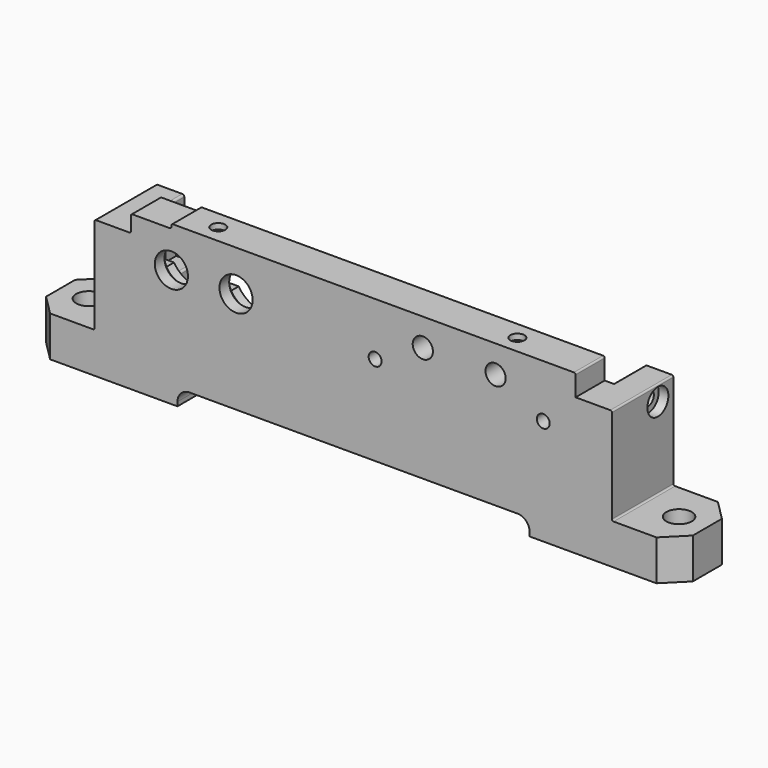
from build123d import *

# Parameters (mm, degrees)
F2_DEPTH     = 9
F3_DEPTH     = 10
F4_R         = 4.1
F4_R_2       = 2.5
F4_R_3       = 1.6
F5_DEPTH     = 24.8
F6_DEPTH     = 3
F4_R_4       = 5
F7_DEPTH     = 6
F4_R_5       = 7.75
F8_DEPTH     = 5
F9_R         = 1.75
F10_DEPTH    = 158.2
F9_R_2       = 3.25
F11_DEPTH    = 2.4
F12_R        = 3.25
F13_DEPTH    = 2.4
F14_R        = 3.4
F14_R_2      = 1.75
F15_DEPTH    = 3
F16_DEPTH    = 25
F17_W        = 100
F17_H        = 9
F18_DEPTH    = 1.1
F20_START    = -1.4
F19_R        = 1.75
F20_DEPTH    = 2.6
F21_DEPTH    = 4.2
F22_W        = 6.7549981495
F22_H        = 2.6
F23_DEPTH    = 4.5
F24_W        = 19
F24_H        = 10
F25_DEPTH    = 16
F26_SIZE     = 5
F27_W        = 19
F27_H        = 10
F28_DEPTH    = 16
F29_SIZE     = 5
F30_R        = 3.15
F31_DEPTH    = 25
F32_R        = 0.4
F33_W        = 87.1225009252
F33_H        = 9
F34_DEPTH    = 4
F35_T1_DEPTH = 9
F37_DEPTH    = 4


# Not quite as in the source:
# - a fillet or chamfer that OpenCascade refuses, or shapes differently, is made with other operations: its cross-section is extruded or revolved along the edge and cut away or added


with BuildPart() as f2:
    # F1 (on face) → F2 (new body)
    with BuildSketch(Plane.XZ):
        Polygon((-55, 28), (-64, 28), (-64, -6), (0, -6), (64, -6), (64, 28), (55, 28), (55, 32.2), (0, 32.2), (-55, 32.2), align=None)
    extrude(amount=F2_DEPTH)

    # F0 (on Front) → F3 (join)
    with BuildSketch(Plane.XZ):
        with BuildLine():
            Line((-57.5, 28), (-64, 28))
            Line((-64, 28), (-64, -6))
            Line((-64, -6), (-43.5, -6))
            Line((-43.5, -6), (-43.5, 0))
            Line((-43.5, 0), (-55, 0))
            ThreePointArc((-55, 0), (-55.3535533906, -0.1464466094), (-55.5, -0.5))
            Line((-55.5, -0.5), (-55.5, -1.5))
            Line((-55.5, -1.5), (-59, -1.5))
            Line((-59, -1.5), (-59, 6.5))
            Line((-59, 6.5), (-54.7, 6.5))
            ThreePointArc((-54.7, 6.5), (-54.3464466094, 6.6464466094), (-54.2, 7))
            Line((-54.2, 7), (-54.2, 13.5))
            ThreePointArc((-54.2, 13.5), (-54.3464466094, 13.8535533906), (-54.7, 14))
            Line((-54.7, 14), (-59, 14))
            Line((-59, 14), (-59, 20.5))
            Line((-59, 20.5), (-57.5, 20.5))
            ThreePointArc((-57.5, 20.5), (-57.1464466094, 20.6464466094), (-57, 21))
            Line((-57, 21), (-57, 27.5))
            ThreePointArc((-57, 27.5), (-57.1464466094, 27.8535533906), (-57.5, 28))
        make_face()
        with BuildLine():
            Line((43.5, -6), (64, -6))
            Line((64, -6), (64, 28))
            Line((64, 28), (57.5, 28))
            ThreePointArc((57.5, 28), (57.1464466094, 27.8535533906), (57, 27.5))
            Line((57, 27.5), (57, 21))
            ThreePointArc((57, 21), (57.1464466094, 20.6464466094), (57.5, 20.5))
            Line((57.5, 20.5), (59, 20.5))
            Line((59, 20.5), (59, 14))
            Line((59, 14), (54.7, 14))
            ThreePointArc((54.7, 14), (54.3464466094, 13.8535533906), (54.2, 13.5))
            Line((54.2, 13.5), (54.2, 7))
            ThreePointArc((54.2, 7), (54.3464466094, 6.6464466094), (54.7, 6.5))
            Line((54.7, 6.5), (59, 6.5))
            Line((59, 6.5), (59, -1.5))
            Line((59, -1.5), (55.5, -1.5))
            Line((55.5, -1.5), (55.5, -0.5))
            ThreePointArc((55.5, -0.5), (55.3535533906, -0.1464466094), (55, 0))
            Line((55, 0), (43.5, 0))
            Line((43.5, 0), (43.5, -6))
        make_face()
    extrude(amount=-F3_DEPTH)

    # F4 (on Front) → F5 (cut)
    with BuildSketch(Plane.XZ):
        with Locations((-29, 23.2)):
            Circle(F4_R)
        with Locations((-45, 23.2)):
            Circle(F4_R)
        with Locations((35.2, 26.5)):
            Circle(F4_R_2)
        with Locations((17.2, 26.5)):
            Circle(F4_R_2)
        with Locations((5.4, 20.2)):
            Circle(F4_R_3)
        with Locations((47, 20.2)):
            Circle(F4_R_3)
    extrude(amount=F5_DEPTH, mode=Mode.SUBTRACT)

    # F4 (on Front) → F6 (cut)
    with BuildSketch(Plane.XZ):
        Polygon((3.7112504626, 17.275), (7.0887495374, 17.275), (8.7774990748, 20.2), (7.0887495374, 23.125), (3.7112504626, 23.125), (2.0225009252, 20.2), align=None)
        with Locations((5.4, 20.2)):
            Circle(F4_R_3, mode=Mode.SUBTRACT)
        Polygon((45.3112504626, 17.275), (48.6887495374, 17.275), (50.3774990748, 20.2), (48.6887495374, 23.125), (45.3112504626, 23.125), (43.6225009252, 20.2), align=None)
        with Locations((47, 20.2)):
            Circle(F4_R_3, mode=Mode.SUBTRACT)
    extrude(amount=F6_DEPTH, mode=Mode.SUBTRACT)

    # F4 (on Front) → F7 (cut)
    with BuildSketch(Plane.XZ):
        with Locations((-45, 23.2)):
            Circle(F4_R_4)
        with Locations((-45, 23.2)):
            Circle(F4_R, mode=Mode.SUBTRACT)
        with Locations((-29, 23.2)):
            Circle(F4_R_4)
        with Locations((-29, 23.2)):
            Circle(F4_R, mode=Mode.SUBTRACT)
    extrude(amount=F7_DEPTH, mode=Mode.SUBTRACT)

    # F4 (on Front) → F8 (cut)
    with BuildSketch(Plane.XZ):
        with Locations((-29, 23.2)):
            Circle(F4_R_5)
        with Locations((-29, 23.2)):
            Circle(F4_R_4, mode=Mode.SUBTRACT)
        with Locations((-45, 23.2)):
            Circle(F4_R_5)
        with Locations((-45, 23.2)):
            Circle(F4_R_4, mode=Mode.SUBTRACT)
    extrude(amount=F8_DEPTH, mode=Mode.SUBTRACT)

    # F9 (on face) → F10 (cut)
    with BuildSketch(Plane(origin=(-64, 0, 0), x_dir=(0, -1, 0), z_dir=(-1, 0, 0))):
        with Locations((-5.2, 24.2)):
            Circle(F9_R)
    extrude(amount=-F10_DEPTH, mode=Mode.SUBTRACT)

    # F9 (on face) → F11 (cut)
    with BuildSketch(Plane(origin=(-64, 0, 0), x_dir=(0, -1, 0), z_dir=(-1, 0, 0))):
        with Locations((-5.2, 24.2)):
            Circle(F9_R_2)
        with Locations((-5.2, 24.2)):
            Circle(F9_R, mode=Mode.SUBTRACT)
    extrude(amount=-F11_DEPTH, mode=Mode.SUBTRACT)

    # F12 (on face) → F13 (cut)
    with BuildSketch(Plane.YZ.offset(64)):
        with Locations((5.2, 24.2)):
            Circle(F12_R)
    extrude(amount=-F13_DEPTH, mode=Mode.SUBTRACT)

    # F14 (on face) → F15 (cut)
    with BuildSketch(Plane(origin=(0, 0, -6), x_dir=(1, 0, 0), z_dir=(0, 0, -1))):
        with Locations((49.8, -5.1)):
            Circle(F14_R)
        with Locations((49.8, -5.1)):
            Circle(F14_R_2, mode=Mode.SUBTRACT)
        with Locations((-48.5, -5.1)):
            Circle(F14_R)
        with Locations((-48.5, -5.1)):
            Circle(F14_R_2, mode=Mode.SUBTRACT)
        with Locations((49.8, -5.1)):
            Circle(F14_R_2)
    extrude(amount=-F15_DEPTH, mode=Mode.SUBTRACT)

    # F14 (on face) → F16 (cut)
    with BuildSketch(Plane(origin=(0, 0, -6), x_dir=(1, 0, 0), z_dir=(0, 0, -1))):
        with Locations((49.8, -5.1)):
            Circle(F14_R_2)
        with Locations((-48.5, -5.1)):
            Circle(F14_R_2)
    extrude(amount=-F16_DEPTH, mode=Mode.SUBTRACT)

    # F17 (on face) → F18 (join)
    with BuildSketch(Plane.XY.offset(32.2)):
        with Locations((5, -4.5)):
            Rectangle(F17_W, F17_H)
    extrude(amount=F18_DEPTH)

    # F19 (on face) → F20 (cut)
    with BuildSketch(Plane.XY.offset(33.3).offset(F20_START)):
        Polygon((35.3112504626, -7.425), (38.6887495374, -7.425), (40.3774990748, -4.5), (38.6887495374, -1.575), (35.3112504626, -1.575), (33.6225009252, -4.5), align=None)
        with Locations((37, -4.5)):
            Circle(F19_R, mode=Mode.SUBTRACT)
        Polygon((-38.6887495374, -7.425), (-35.3112504626, -7.425), (-33.6225009252, -4.5), (-35.3112504626, -1.575), (-38.6887495374, -1.575), (-40.3774990748, -4.5), align=None)
        with Locations((-37, -4.5)):
            Circle(F19_R, mode=Mode.SUBTRACT)
    extrude(amount=-F20_DEPTH, mode=Mode.SUBTRACT)

    # F19 (on face) → F21 (cut)
    with BuildSketch(Plane.XY.offset(33.3)):
        with Locations((-37, -4.5)):
            Circle(F19_R)
        with Locations((37, -4.5)):
            Circle(F19_R)
    extrude(amount=-F21_DEPTH, mode=Mode.SUBTRACT)

    # F22 (on face) → F23 (cut)
    with BuildSketch(Plane(origin=(0, 0, 0), x_dir=(-1, 0, 0), z_dir=(0, 1, 0))):
        with Locations((-37, 30.6)):
            Rectangle(F22_W, F22_H)
        with Locations((37, 30.6)):
            Rectangle(F22_W, F22_H)
    extrude(amount=-F23_DEPTH, mode=Mode.SUBTRACT)

    # F24 (on face) → F25 (join)
    with BuildSketch(Plane(origin=(-64, 0, 0), x_dir=(0, -1, 0), z_dir=(-1, 0, 0))):
        with Locations((-0.5, -1)):
            Rectangle(F24_W, F24_H)
    extrude(amount=F25_DEPTH)

    # F26
    f26_edges = [f2.edges().sort_by_distance(p)[0] for p in [
        (-80, -9, -1),
        (-80, 10, -1),
    ]]
    chamfer(f26_edges, length=F26_SIZE)

    # F27 (on face) → F28 (join)
    with BuildSketch(Plane.YZ.offset(64)):
        with Locations((0.5, -1)):
            Rectangle(F27_W, F27_H)
    extrude(amount=F28_DEPTH)

    # F29
    f29_edges = [f2.edges().sort_by_distance(p)[0] for p in [
        (80, 10, -1),
        (80, -9, -1),
    ]]
    chamfer(f29_edges, length=F29_SIZE)

    # F30 (on face) → F31 (cut)
    with BuildSketch(Plane(origin=(0, 0, -6), x_dir=(1, 0, 0), z_dir=(0, 0, -1))):
        with Locations((-73, -0.5)):
            Circle(F30_R)
        with Locations((73, -0.5)):
            Circle(F30_R)
    extrude(amount=-F31_DEPTH, mode=Mode.SUBTRACT)

    # F32
    f32_edges = [f2.edges().sort_by_distance(p)[0] for p in [
        (64, 0.5, 28),
        (55, -4.5, 33.3),
        (-64, 0.5, 28),
        (-55, -4.5, 28),
        (-55, -4.5, 32.2),
        (-45, -4.5, 32.2),
        (-45, -4.5, 33.3),
        (-64, 0.5, 4),
        (64, 0.5, 4),
    ]]
    fillet(f32_edges, radius=F32_R)

    # F33 (on face) → F34 (cut)
    with BuildSketch(Plane(origin=(0, 0, -6), x_dir=(1, 0, 0), z_dir=(0, 0, -1))):
        with Locations((0.0612504626, 4.5)):
            Rectangle(F33_W, F33_H)
    extrude(amount=-F34_DEPTH, mode=Mode.SUBTRACT)

    # F35: fillet of radius 3 on 2 edges, made by hand

    # F35_s2 → F35_t1 (join)
    with BuildSketch(Plane.XZ):
        with BuildLine():
            ThreePointArc((-43.5, -5), (-42.6213203436, -2.8786796564), (-40.5, -2))
            Line((-40.5, -2), (-43.5, -2))
            Line((-43.5, -2), (-43.5, -5))
        make_face()
        with BuildLine():
            ThreePointArc((40.6225009252, -2), (42.7438212688, -2.8786796564), (43.6225009252, -5))
            Line((43.6225009252, -5), (43.6225009252, -2))
            Line((43.6225009252, -2), (40.6225009252, -2))
        make_face()
    extrude(amount=F35_T1_DEPTH)

    # F36 (on face) → F37 (cut)
    with BuildSketch(Plane(origin=(0, 0, 0), x_dir=(-1, 0, 0), z_dir=(0, 1, 0))):
        with BuildLine():
            Line((22.4636435891, 27.3639578372), (19.415192306, 27.3639578372))
            Line((19.415192306, 27.3639578372), (19.415192306, 19.0618205816))
            Line((19.415192306, 19.0618205816), (22.4472928418, 19.0618205816))
            ThreePointArc((22.4472928418, 19.0618205816), (21.5553381381, 21.0460478738), (21.25, 23.2))
            ThreePointArc((21.25, 23.2), (21.5595946957, 25.3686099022), (22.4636435891, 27.3639578372))
        make_face()
        with BuildLine():
            Line((38.4636435891, 27.3639578372), (35.5363564109, 27.3639578372))
            ThreePointArc((35.5363564109, 27.3639578372), (36.7499849698, 23.2152633041), (35.5527071582, 19.0618205816))
            Line((35.5527071582, 19.0618205816), (38.4472928418, 19.0618205816))
            ThreePointArc((38.4472928418, 19.0618205816), (37.5553381381, 21.0460478738), (37.25, 23.2))
            ThreePointArc((37.25, 23.2), (37.5595946957, 25.3686099022), (38.4636435891, 27.3639578372))
        make_face()
        with BuildLine():
            Line((53.6553673446, 27.3639578372), (51.5363564109, 27.3639578372))
            ThreePointArc((51.5363564109, 27.3639578372), (52.7499849698, 23.2152633041), (51.5527071582, 19.0618205816))
            Line((51.5527071582, 19.0618205816), (53.6553673446, 19.0618205816))
            Line((53.6553673446, 19.0618205816), (53.6553673446, 27.3639578372))
        make_face()
    extrude(amount=-F37_DEPTH, mode=Mode.SUBTRACT)


solid = f2.part
